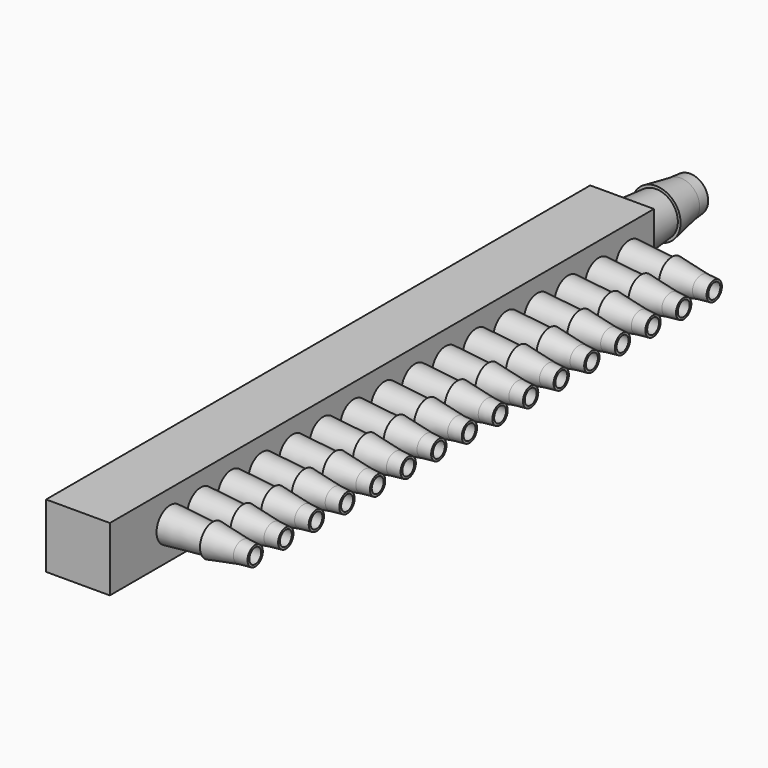
from build123d import *

# Parameters (mm, degrees)
F1_W           = 19.05
F1_H           = 19.05
F2_DEPTH       = 203.2
F0_R           = 6.35
F3_DEPTH       = 190.5
F4_R           = 5.08
F6_DEPTH       = 25.4
F6_TAPER       = 5
F7_R           = 7.62
F8_DEPTH       = 25.4
F8_TAPER       = 5
F10_R          = 5.08
F11_DEPTH      = 12.7
F11_TAPER      = -10
F9_R           = 4.445
F12_DEPTH      = 27.94
F12_TAPER      = -5
F13_R          = 2.54
F14_DEPTH      = 12.7
F14_TAPER      = -10
F5_R           = 4.445
F15_DEPTH      = 25.4
F15_TAPER      = 5
F15_DEPTH_BACK = 12.7


with BuildPart() as f2:
    # F1 (on Front) → F2 (new body)
    with BuildSketch(Plane.XZ):
        Rectangle(F1_W, F1_H)
    extrude(amount=F2_DEPTH)

    # F0 (on Front) → F3 (cut)
    with BuildSketch(Plane.XZ):
        Circle(F0_R)
    extrude(amount=F3_DEPTH, mode=Mode.SUBTRACT)

    # F4 (on face) → F6 (join)
    with BuildSketch(Plane.YZ.offset(9.525)):
        with Locations((-9.2296069488, 0)):
            Circle(F4_R)
        with Locations((-20.6596069488, 0)):
            Circle(F4_R)
        with Locations((-32.0896069488, 0)):
            Circle(F4_R)
        with Locations((-43.5196069488, 0)):
            Circle(F4_R)
        with Locations((-54.9496069488, 0)):
            Circle(F4_R)
        with Locations((-66.3796069488, 0)):
            Circle(F4_R)
        with Locations((-77.8096069488, 0)):
            Circle(F4_R)
        with Locations((-89.2396069488, 0)):
            Circle(F4_R)
        with Locations((-100.6696069488, 0)):
            Circle(F4_R)
        with Locations((-112.0996069488, 0)):
            Circle(F4_R)
        with Locations((-123.5296069488, 0)):
            Circle(F4_R)
        with Locations((-134.9596069488, 0)):
            Circle(F4_R)
        with Locations((-146.3896069488, 0)):
            Circle(F4_R)
        with Locations((-157.8196069488, 0)):
            Circle(F4_R)
        with Locations((-169.2496069488, 0)):
            Circle(F4_R)
        with Locations((-180.6796069488, 0)):
            Circle(F4_R)
    extrude(amount=F6_DEPTH, taper=F6_TAPER)

    # F7 (on face) → F8 (join)
    with BuildSketch(Plane(origin=(0, 0, 0), x_dir=(-1, 0, 0), z_dir=(0, 1, 0))):
        Circle(F7_R)
    extrude(amount=F8_DEPTH, taper=F8_TAPER)

    # F10 (on face) → F11 (join)
    with BuildSketch(Plane(origin=(0, 25.4, 0), x_dir=(-1, 0, 0), z_dir=(0, 1, 0))):
        Circle(F10_R)
    extrude(amount=-F11_DEPTH, taper=F11_TAPER)

    # F9 (on face) → F12 (cut)
    with BuildSketch(Plane(origin=(0, 25.4, 0), x_dir=(-1, 0, 0), z_dir=(0, 1, 0))):
        Circle(F9_R)
    extrude(amount=-F12_DEPTH, taper=F12_TAPER, mode=Mode.SUBTRACT)

    # F13 (on face) → F14 (join)
    with BuildSketch(Plane.YZ.offset(34.925)):
        with Locations((-9.1966530308, 0)):
            Circle(F13_R)
        with Locations((-20.6266530308, 0)):
            Circle(F13_R)
        with Locations((-32.0566530308, 0)):
            Circle(F13_R)
        with Locations((-43.4866530308, 0)):
            Circle(F13_R)
        with Locations((-54.9166530308, 0)):
            Circle(F13_R)
        with Locations((-66.3466530308, 0)):
            Circle(F13_R)
        with Locations((-77.7766530308, 0)):
            Circle(F13_R)
        with Locations((-89.2066530308, 0)):
            Circle(F13_R)
        with Locations((-100.6366530308, 0)):
            Circle(F13_R)
        with Locations((-112.0666530308, 0)):
            Circle(F13_R)
        with Locations((-123.4966530308, 0)):
            Circle(F13_R)
        with Locations((-134.9266530308, 0)):
            Circle(F13_R)
        with Locations((-146.3566530308, 0)):
            Circle(F13_R)
        with Locations((-157.7866530308, 0)):
            Circle(F13_R)
        with Locations((-169.2166530308, 0)):
            Circle(F13_R)
        with Locations((-180.6466530308, 0)):
            Circle(F13_R)
    extrude(amount=-F14_DEPTH, taper=F14_TAPER)

    # F5 (on face) → F15 (cut, two sides)
    with BuildSketch(Plane.YZ.offset(9.525)) as f15_sk:
        with Locations((-9.1966530308, 0)):
            Circle(F5_R)
        with Locations((-20.6266530308, 0)):
            Circle(F5_R)
        with Locations((-32.0566530308, 0)):
            Circle(F5_R)
        with Locations((-43.4866530308, 0)):
            Circle(F5_R)
        with Locations((-54.9166530308, 0)):
            Circle(F5_R)
        with Locations((-66.3466530308, 0)):
            Circle(F5_R)
        with Locations((-77.7766530308, 0)):
            Circle(F5_R)
        with Locations((-89.2066530308, 0)):
            Circle(F5_R)
        with Locations((-100.6366530308, 0)):
            Circle(F5_R)
        with Locations((-112.0666530308, 0)):
            Circle(F5_R)
        with Locations((-123.4966530308, 0)):
            Circle(F5_R)
        with Locations((-134.9266530308, 0)):
            Circle(F5_R)
        with Locations((-146.3566530308, 0)):
            Circle(F5_R)
        with Locations((-157.7866530308, 0)):
            Circle(F5_R)
        with Locations((-169.2166530308, 0)):
            Circle(F5_R)
        with Locations((-180.6466530308, 0)):
            Circle(F5_R)
    extrude(amount=F15_DEPTH, taper=F15_TAPER, mode=Mode.SUBTRACT)
    extrude(f15_sk.sketch, amount=-F15_DEPTH_BACK, mode=Mode.SUBTRACT)


solid = f2.part
